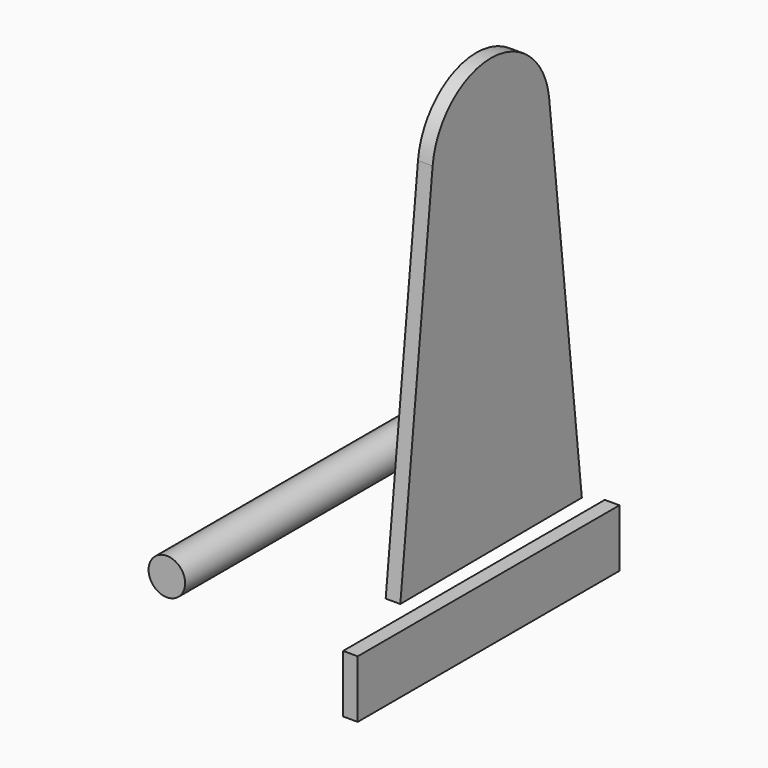
from build123d import *

# Parameters (mm, degrees)
F0_R     = 3.175
F1_DEPTH = 56.769
F2_W     = 56.7667558789
F2_H     = 10.0242104381
F3_DEPTH = 2.54
F5_DEPTH = 2.54


# Not quite as in the source:
# - a feature names something its author has since deleted; it is built from what else it names


with BuildPart() as f1:
    # F0 (on Front) → F1 (new body)
    with BuildSketch(Plane.XZ):
        with Locations((-30.5883418769, 27.933979407)):
            Circle(F0_R)
    extrude(amount=F1_DEPTH)


with BuildPart() as f3:
    # F2 (on Right) → F3 (new body)
    with BuildSketch(Plane.YZ):
        with Locations((-28.3833779395, 21.5122671798)):
            Rectangle(F2_W, F2_H)
    extrude(amount=F3_DEPTH)


with BuildPart() as f5:
    # F4 (on Right) → F5 (new body)
    with BuildSketch(Plane.YZ):
        with BuildLine():
            ThreePointArc((-15.2336207801, 94.8577174533), (-15.1755603882, 94.1580515789), (-15.1561872556, 93.4562481686))
            ThreePointArc((-15.1561872556, 93.4562481686), (-28.570028053, 80.7537998705), (-40.5234116559, 94.8392511643))
            Line((-40.5234116559, 94.8392511643), (-47.5317611003, 30.7562586925))
            Line((-47.5317611003, 30.7562586925), (-8.1549498937, 30.9948429335))
            Line((-8.1549498937, 30.9948429335), (-15.2336207801, 94.8577174533))
        make_face()
        with BuildLine():
            ThreePointArc((-40.5234116559, 94.8392511643), (-28.570028053, 80.7537998705), (-15.1561872556, 93.4562481686))
            ThreePointArc((-15.1561872556, 93.4562481686), (-15.1755603882, 94.1580515789), (-15.2336207801, 94.8577174533))
            ThreePointArc((-15.2336207801, 94.8577174533), (-27.8867885653, 106.1775571463), (-40.5234116559, 94.8392511643))
        make_face()
    extrude(amount=F5_DEPTH)


solid = Compound([f1.part, f3.part, f5.part])
